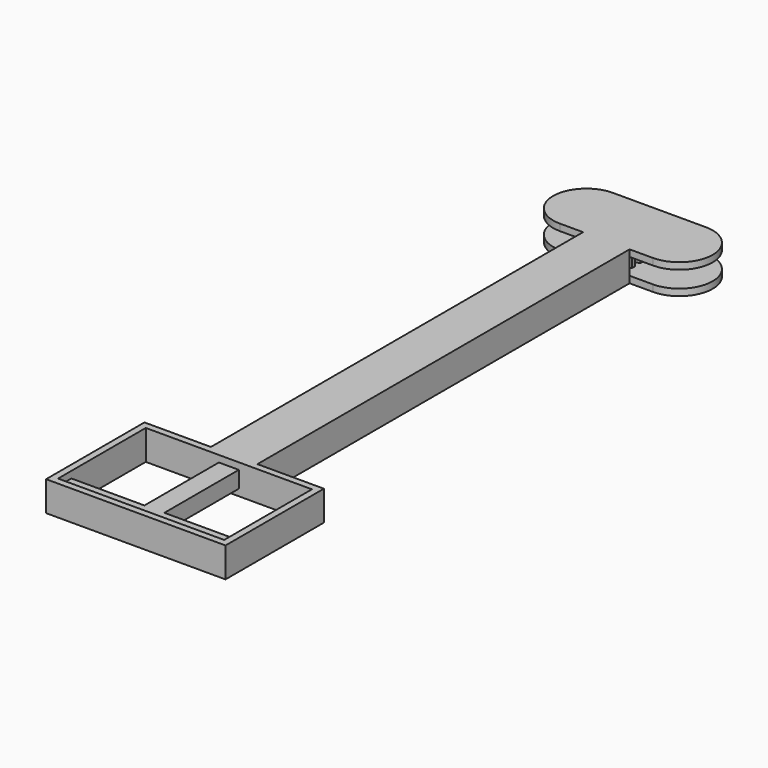
from build123d import *

# Parameters (mm, degrees)
F1_DEPTH      = 5
F3_W          = 50
F3_H          = 5
F4_DEPTH      = 5
F5_W          = 50
F5_H          = 33
F6_DEPTH      = 7
F6_DEPTH_BACK = 2
F9_DEPTH      = 5
F10_W         = 10
F10_H         = 5
F11_DEPTH     = 50


with BuildPart() as f1:
    # F0 (on Top) → F1 (new body)
    with BuildSketch(Plane.XY):
        Polygon((3, 13), (0, 13), (0, -180), (3, -180), (3, -39.0871235167), (3, -36.9128764833), (3, -35.8871235167), (3, -33.7128764833), (3, -32.6871235167), (3, -30.5128764833), (3, -29.4871235167), (3, -27.3128764833), (3, -26.2871235167), (3, -24.1128764833), (3, -23.0871235167), (3, -20.9128764833), (3, -19.8871235167), (3, -17.7128764833), (3, -16.6871235167), (3, -14.5128764833), (3, -13.4871235167), (3, -11.3128764833), (3, -10.2871235167), (3, -8.1128764833), (3, -7.0871235167), (3, -4.9128764833), (3, -3.8871235167), (3, -1.7128764833), (3, -0.6871235167), (3, 1.4871235167), (3, 2.5128764833), (3, 4.6871235167), (3, 5.7128764833), (3, 7.8871235167), (3, 8.9128764833), (3, 11.0871235167), align=None)
        with BuildLine():
            ThreePointArc((5, 10.5), (4.0421988802, 10.9373096378), (3, 11.0871235167))
            Line((3, 11.0871235167), (3, 8.9128764833))
            ThreePointArc((3, 8.9128764833), (4.0421988802, 9.0626903622), (5, 9.5))
            Line((5, 9.5), (5, 10))
            Line((5, 10), (5, 10.5))
        make_face()
        with BuildLine():
            Line((3, -36.9128764833), (3, -39.0871235167))
            ThreePointArc((3, -39.0871235167), (4.0421988802, -38.9373096378), (5, -38.5))
            Line((5, -38.5), (5, -38))
            Line((5, -38), (5, -37.5))
            ThreePointArc((5, -37.5), (4.0421988802, -37.0626903622), (3, -36.9128764833))
        make_face()
        with BuildLine():
            ThreePointArc((5, 7.3), (4.0421988802, 7.7373096378), (3, 7.8871235167))
            Line((3, 7.8871235167), (3, 5.7128764833))
            ThreePointArc((3, 5.7128764833), (4.0421988802, 5.8626903622), (5, 6.3))
            Line((5, 6.3), (5, 6.8))
            Line((5, 6.8), (5, 7.3))
        make_face()
        with BuildLine():
            Line((3, -33.7128764833), (3, -35.8871235167))
            ThreePointArc((3, -35.8871235167), (4.0421988802, -35.7373096378), (5, -35.3))
            Line((5, -35.3), (5, -34.8))
            Line((5, -34.8), (5, -34.3))
            ThreePointArc((5, -34.3), (4.0421988802, -33.8626903622), (3, -33.7128764833))
        make_face()
        with BuildLine():
            ThreePointArc((5, 4.1), (4.0421988802, 4.5373096378), (3, 4.6871235167))
            Line((3, 4.6871235167), (3, 2.5128764833))
            ThreePointArc((3, 2.5128764833), (4.0421988802, 2.6626903622), (5, 3.1))
            Line((5, 3.1), (5, 3.6))
            Line((5, 3.6), (5, 4.1))
        make_face()
        with BuildLine():
            Line((3, -30.5128764833), (3, -32.6871235167))
            ThreePointArc((3, -32.6871235167), (4.0421988802, -32.5373096378), (5, -32.1))
            Line((5, -32.1), (5, -31.6))
            Line((5, -31.6), (5, -31.1))
            ThreePointArc((5, -31.1), (4.0421988802, -30.6626903622), (3, -30.5128764833))
        make_face()
        with BuildLine():
            ThreePointArc((5, 0.9), (4.0421988802, 1.3373096378), (3, 1.4871235167))
            Line((3, 1.4871235167), (3, -0.6871235167))
            ThreePointArc((3, -0.6871235167), (4.0421988802, -0.5373096378), (5, -0.1))
            Line((5, -0.1), (5, 0.4))
            Line((5, 0.4), (5, 0.9))
        make_face()
        with BuildLine():
            Line((3, -27.3128764833), (3, -29.4871235167))
            ThreePointArc((3, -29.4871235167), (4.0421988802, -29.3373096378), (5, -28.9))
            Line((5, -28.9), (5, -28.4))
            Line((5, -28.4), (5, -27.9))
            ThreePointArc((5, -27.9), (4.0421988802, -27.4626903622), (3, -27.3128764833))
        make_face()
        with BuildLine():
            ThreePointArc((5, -2.3), (4.0421988802, -1.8626903622), (3, -1.7128764833))
            Line((3, -1.7128764833), (3, -3.8871235167))
            ThreePointArc((3, -3.8871235167), (4.0421988802, -3.7373096378), (5, -3.3))
            Line((5, -3.3), (5, -2.8))
            Line((5, -2.8), (5, -2.3))
        make_face()
        with BuildLine():
            Line((3, -24.1128764833), (3, -26.2871235167))
            ThreePointArc((3, -26.2871235167), (4.0421988802, -26.1373096378), (5, -25.7))
            Line((5, -25.7), (5, -25.2))
            Line((5, -25.2), (5, -24.7))
            ThreePointArc((5, -24.7), (4.0421988802, -24.2626903622), (3, -24.1128764833))
        make_face()
        with BuildLine():
            ThreePointArc((5, -5.5), (4.0421988802, -5.0626903622), (3, -4.9128764833))
            Line((3, -4.9128764833), (3, -7.0871235167))
            ThreePointArc((3, -7.0871235167), (4.0421988802, -6.9373096378), (5, -6.5))
            Line((5, -6.5), (5, -6))
            Line((5, -6), (5, -5.5))
        make_face()
        with BuildLine():
            Line((3, -20.9128764833), (3, -23.0871235167))
            ThreePointArc((3, -23.0871235167), (4.0421988802, -22.9373096378), (5, -22.5))
            Line((5, -22.5), (5, -22))
            Line((5, -22), (5, -21.5))
            ThreePointArc((5, -21.5), (4.0421988802, -21.0626903622), (3, -20.9128764833))
        make_face()
        with BuildLine():
            ThreePointArc((5, -8.7), (4.0421988802, -8.2626903622), (3, -8.1128764833))
            Line((3, -8.1128764833), (3, -10.2871235167))
            ThreePointArc((3, -10.2871235167), (4.0421988802, -10.1373096378), (5, -9.7))
            Line((5, -9.7), (5, -9.2))
            Line((5, -9.2), (5, -8.7))
        make_face()
        with BuildLine():
            Line((3, -17.7128764833), (3, -19.8871235167))
            ThreePointArc((3, -19.8871235167), (4.0421988802, -19.7373096378), (5, -19.3))
            Line((5, -19.3), (5, -18.8))
            Line((5, -18.8), (5, -18.3))
            ThreePointArc((5, -18.3), (4.0421988802, -17.8626903622), (3, -17.7128764833))
        make_face()
        with BuildLine():
            ThreePointArc((5, -11.9), (4.0421988802, -11.4626903622), (3, -11.3128764833))
            Line((3, -11.3128764833), (3, -13.4871235167))
            ThreePointArc((3, -13.4871235167), (4.0421988802, -13.3373096378), (5, -12.9))
            Line((5, -12.9), (5, -12.4))
            Line((5, -12.4), (5, -11.9))
        make_face()
        with BuildLine():
            Line((3, -14.5128764833), (3, -16.6871235167))
            ThreePointArc((3, -16.6871235167), (4.0421988802, -16.5373096378), (5, -16.1))
            Line((5, -16.1), (5, -15.6))
            Line((5, -15.6), (5, -15.1))
            ThreePointArc((5, -15.1), (4.0421988802, -14.6626903622), (3, -14.5128764833))
        make_face()
    extrude(amount=F1_DEPTH)

    # F2: F1 across face


with BuildPart() as f1_1:
    add(f1.part)
    add(f1.part.mirror(Plane(origin=(0, -83.5, 2.5), x_dir=(0, -1, 0), z_dir=(-1, 0, 0))))

    # F3 (on face) → F4 (join)
    with BuildSketch(Plane.XZ.offset(180)):
        with Locations((0, 2.5)):
            Rectangle(F3_W, F3_H)
    extrude(amount=F4_DEPTH)


with BuildPart() as f6:
    # F5 (on Top) → F6 (new body, two sides)
    with BuildSketch(Plane.XY) as f6_sk:
        with BuildLine():
            ThreePointArc((14, -10), (21.0710678119, -7.0710678119), (24, 0))
            ThreePointArc((24, 0), (21.0710678119, 7.0710678119), (14, 10))
            ThreePointArc((14, 10), (4, 0), (14, -10))
        make_face()
        with BuildLine():
            ThreePointArc((14, -10), (4, 0), (14, 10))
            Line((14, 10), (0, 10))
            Line((0, 10), (-14, 10))
            ThreePointArc((-14, 10), (-6.9289321881, 7.0710678119), (-4, 0))
            ThreePointArc((-4, 0), (-6.9289321881, -7.0710678119), (-14, -10))
            Line((-14, -10), (-7, -10))
            Line((-7, -10), (-7, -150))
            Line((-7, -150), (-27, -150))
            Line((-27, -150), (-27, -187))
            Line((-27, -187), (0, -187))
            Line((0, -187), (27, -187))
            Line((27, -187), (27, -150))
            Line((27, -150), (7, -150))
            Line((7, -150), (7, -10))
            Line((7, -10), (14, -10))
        make_face()
        with Locations((0, -168.5)):
            Rectangle(F5_W, F5_H, mode=Mode.SUBTRACT)
        with BuildLine():
            ThreePointArc((-4, 0), (-6.9289321881, 7.0710678119), (-14, 10))
            ThreePointArc((-14, 10), (-24, 0), (-14, -10))
            ThreePointArc((-14, -10), (-6.9289321881, -7.0710678119), (-4, 0))
        make_face()
    extrude(amount=F6_DEPTH)
    extrude(f6_sk.sketch, amount=-F6_DEPTH_BACK)

    # F7: cut F1
    add(f1_1.part, mode=Mode.SUBTRACT)

    # F8 (on Top) → F9 (cut)
    with BuildSketch(Plane.XY):
        with BuildLine():
            ThreePointArc((-14, 10), (-24, 0), (-14, -10))
            Line((-14, -10), (14, -10))
            ThreePointArc((14, -10), (24, 0), (14, 10))
            Line((14, 10), (-14, 10))
        make_face()
    extrude(amount=F9_DEPTH, mode=Mode.SUBTRACT)

    # F10 (on face) → F11 (cut)
    with BuildSketch(Plane(origin=(0, -10, 0), x_dir=(-1, 0, 0), z_dir=(0, 1, 0))):
        with Locations((0, 2.5)):
            Rectangle(F10_W, F10_H)
    extrude(amount=-F11_DEPTH, mode=Mode.SUBTRACT)


solid = Compound([f1_1.part, f6.part])
